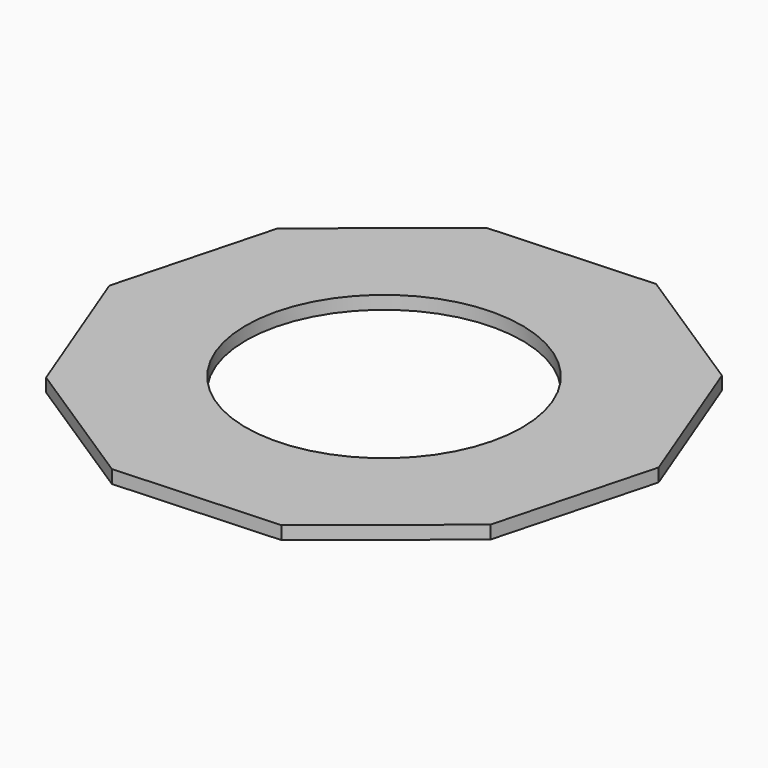
from build123d import *

# Parameters (mm, degrees)
F3_DEPTH = 2.54
F4_R     = 26.6451921389
F5_DEPTH = 25.4


# Not quite as in the source:
# - the program builds the solid bodies; features that only make, move or delete a surface that nothing else refers to are left out


with BuildPart() as f3:
    # F0 (on Top) → F3 (new body)
    with BuildSketch(Plane.XY):
        Polygon((13.1522906624, 49.1708465148), (-18.2614717633, 47.5107729435), (-42.69997266, 27.7031989396), (-50.8285353193, -2.6860554622), (-39.542325085, -32.049327973), (-13.1522906624, -49.1708465148), (18.2614717633, -47.5107729435), (42.69997266, -27.7031989396), (50.8285353193, 2.6860554622), (39.542325085, 32.049327973), align=None)
    extrude(amount=F3_DEPTH)

    # F4 (on face) → F5 (cut)
    with BuildSketch(Plane(origin=(0, 0, 0), x_dir=(1, 0, 0), z_dir=(0, 0, -1))):
        Circle(F4_R)
    extrude(amount=-F5_DEPTH, mode=Mode.SUBTRACT)


solid = f3.part
